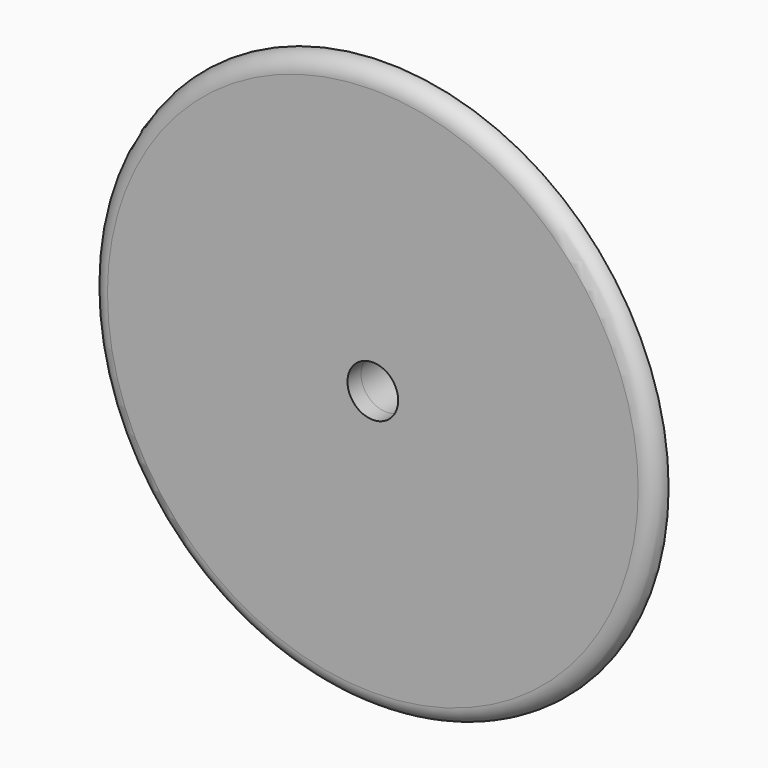
from build123d import *

# Parameters (mm, degrees)
F0_R     = 50.1
F0_R_2   = 4.5
F1_DEPTH = 3
F2_R     = 7.5
F2_R_2   = 4.5
F3_DEPTH = 25
F4_R     = 2.99999


# Not quite as in the source:
# - a fillet or chamfer is up to 0.001 mm smaller than in the source, because OpenCascade refuses the exact size


with BuildPart() as f1:
    # F0 (on Front) → F1 (new body)
    with BuildSketch(Plane.XZ):
        Circle(F0_R)
        Circle(F0_R_2, mode=Mode.SUBTRACT)
    extrude(amount=F1_DEPTH)

    # F2 (on face) → F3 (join)
    with BuildSketch(Plane(origin=(0, 0, 0), x_dir=(-1, 0, 0), z_dir=(0, 1, 0))):
        Circle(F2_R)
        Circle(F2_R_2, mode=Mode.SUBTRACT)
    extrude(amount=F3_DEPTH)

    # F4 (radius 3 in the source; OpenCascade refuses exactly that, so slightly less here)
    f4_edges = [f1.edges().sort_by_distance(p)[0] for p in [
        (-50.1, -3, 0),
    ]]
    fillet(f4_edges, radius=F4_R)


solid = f1.part
